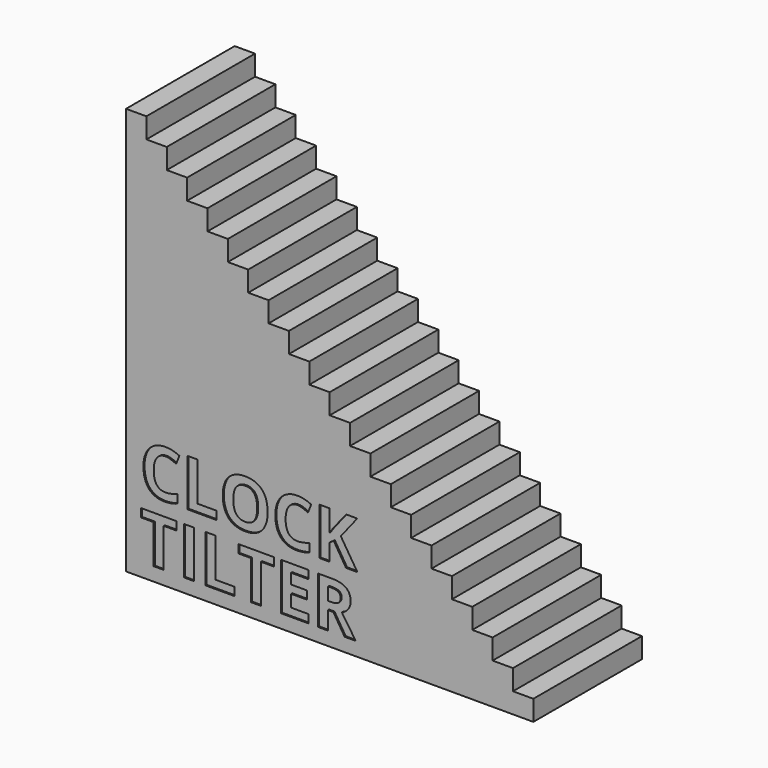
from build123d import *

# Parameters (mm, degrees)
F0_W         = 1.4720052083
F0_H         = 6.9407552083
F0_TEXT_SIZE = 9.7222222222
F1_DEPTH     = 20
F2_DEPTH     = 0.2


# Not quite as in the source:
# - Text() gives the source's letters only with a copy of the font that has no kerning and outlines rounded to 1/6400 em; it was checked with that copy


with BuildPart() as f1:
    # F0 (on Front) → F1 (new body)
    with BuildSketch(Plane.XZ):
        Polygon((-37.6443677493, -13.4150516285), (22.3556322507, -13.4150516285), (22.3556322507, -10.4150516285), (19.3556322507, -10.4150516285), (19.3556322507, -7.4150516285), (16.3556322507, -7.4150516285), (16.3556322507, -4.4150516285), (13.3556322507, -4.4150516285), (13.3556322507, -1.4150516285), (10.3556322507, -1.4150516285), (10.3556322507, 1.5849483715), (7.3556322507, 1.5849483715), (7.3556322507, 4.5849483715), (4.3556322507, 4.5849483715), (4.3556322507, 7.5849483715), (1.3556322507, 7.5849483715), (1.3556322507, 10.5849483715), (-1.6443677493, 10.5849483715), (-1.6443677493, 13.5849483715), (-4.6443677493, 13.5849483715), (-4.6443677493, 16.5849483715), (-7.6443677493, 16.5849483715), (-7.6443677493, 19.5849483715), (-10.6443677493, 19.5849483715), (-10.6443677493, 22.5849483715), (-13.6443677493, 22.5849483715), (-13.6443677493, 25.5849483715), (-16.6443677493, 25.5849483715), (-16.6443677493, 28.5849483715), (-19.6443677493, 28.5849483715), (-19.6443677493, 31.5849483715), (-22.6443677493, 31.5849483715), (-22.6443677493, 34.5849483715), (-25.6443677493, 34.5849483715), (-25.6443677493, 37.5849483715), (-28.6443677493, 37.5849483715), (-28.6443677493, 40.5849483715), (-31.6443677493, 40.5849483715), (-31.6443677493, 43.5849483715), (-34.6443677493, 43.5849483715), (-34.6443677493, 46.5849483715), (-37.6443677493, 46.5849483715), align=None)
        Polygon((-32.0927184437, -5.6986887813), (-32.0927184437, -11.4150516285), (-33.564723652, -11.4150516285), (-33.564723652, -5.6986887813), (-35.4499233048, -5.6986887813), (-35.4499233048, -4.4742964201), (-30.2090378882, -4.4742964201), (-30.2090378882, -5.6986887813), align=None, mode=Mode.SUBTRACT)
        with Locations((-28.4051099368, -7.9446740243)):
            Rectangle(F0_W, F0_H, mode=Mode.SUBTRACT)
        Polygon((-21.6352531659, -11.4150516285), (-25.922145527, -11.4150516285), (-25.922145527, -4.4742964201), (-24.4501403187, -4.4742964201), (-24.4501403187, -10.1997738507), (-21.6352531659, -10.1997738507), align=None, mode=Mode.SUBTRACT)
        with BuildLine():
            add(Edge.make_bspline(
                [(-31.049098652, 3.2625742396), (-31.4425448326, 3.4000525382), (-31.8223191382, 3.4000525382)],
                knots=[0, 0, 0, 1, 1, 1], degree=2))
            add(Edge.make_bspline(
                [(-31.8223191382, 3.4000525382), (-32.6532653187, 3.4000525382), (-33.1089944854, 2.7757035799)],
                knots=[0, 0, 0, 1, 1, 1], degree=2))
            add(Edge.make_bspline(
                [(-33.1089944854, 2.7757035799), (-33.564723652, 2.1513546215), (-33.564723652, 1.0363372604)],
                knots=[0, 0, 0, 1, 1, 1], degree=2))
            add(Edge.make_bspline(
                [(-33.564723652, 1.0363372604), (-33.564723652, -1.2848432951), (-31.8223191382, -1.2848432951)],
                knots=[0, 0, 0, 1, 1, 1], degree=2))
            add(Edge.make_bspline(
                [(-31.8223191382, -1.2848432951), (-31.0916333743, -1.2848432951), (-30.0525708743, -0.9202599618)],
                knots=[0, 0, 0, 1, 1, 1], degree=2))
            Line((-30.0525708743, -0.9202599618), (-30.0525708743, -2.1537669063))
            add(Edge.make_bspline(
                [(-30.0525708743, -2.1537669063), (-30.9063035132, -2.5107547535), (-31.9605569854, -2.5107547535)],
                knots=[0, 0, 0, 1, 1, 1], degree=2))
            add(Edge.make_bspline(
                [(-31.9605569854, -2.5107547535), (-33.4750969159, -2.5107547535), (-34.2771802493, -1.591700934)],
                knots=[0, 0, 0, 1, 1, 1], degree=2))
            add(Edge.make_bspline(
                [(-34.2771802493, -1.591700934), (-35.0792635826, -0.6726471146), (-35.0792635826, 1.0454518437)],
                knots=[0, 0, 0, 1, 1, 1], degree=2))
            add(Edge.make_bspline(
                [(-35.0792635826, 1.0454518437), (-35.0792635826, 2.1285681632), (-34.6850578534, 2.9428042743)],
                knots=[0, 0, 0, 1, 1, 1], degree=2))
            add(Edge.make_bspline(
                [(-34.6850578534, 2.9428042743), (-34.2908521243, 3.7570403854), (-33.5525708743, 4.1907426424)],
                knots=[0, 0, 0, 1, 1, 1], degree=2))
            add(Edge.make_bspline(
                [(-33.5525708743, 4.1907426424), (-32.8142896243, 4.6244448993), (-31.8223191382, 4.6244448993)],
                knots=[0, 0, 0, 1, 1, 1], degree=2))
            add(Edge.make_bspline(
                [(-31.8223191382, 4.6244448993), (-30.8121194854, 4.6244448993), (-29.791286152, 4.136814691)],
                knots=[0, 0, 0, 1, 1, 1], degree=2))
            Line((-29.791286152, 4.136814691), (-30.2652444854, 2.9397660799))
            add(Edge.make_bspline(
                [(-30.2652444854, 2.9397660799), (-30.6556524715, 3.125095941), (-31.049098652, 3.2625742396)],
                knots=[0, 0, 0, 1, 1, 1], degree=2))
        make_face(mode=Mode.SUBTRACT)
        Polygon((-24.2891160132, -2.4150516285), (-28.5760083743, -2.4150516285), (-28.5760083743, 4.5257035799), (-27.1040031659, 4.5257035799), (-27.1040031659, -1.1997738507), (-24.2891160132, -1.1997738507), align=None, mode=Mode.SUBTRACT)
        Polygon((-17.7509215687, -5.6986887813), (-17.7509215687, -11.4150516285), (-19.222926777, -11.4150516285), (-19.222926777, -5.6986887813), (-21.1081264298, -5.6986887813), (-21.1081264298, -4.4742964201), (-15.8672410132, -4.4742964201), (-15.8672410132, -5.6986887813), align=None, mode=Mode.SUBTRACT)
        Polygon((-10.8025708743, -10.1997738507), (-10.8025708743, -11.4150516285), (-14.7993156659, -11.4150516285), (-14.7993156659, -4.4742964201), (-10.8025708743, -4.4742964201), (-10.8025708743, -5.6804596146), (-13.3273104576, -5.6804596146), (-13.3273104576, -7.2041141285), (-10.9772670548, -7.2041141285), (-10.9772670548, -8.4102773229), (-13.3273104576, -8.4102773229), (-13.3273104576, -10.1997738507), align=None, mode=Mode.SUBTRACT)
        with BuildLine():
            add(Edge.make_bspline(
                [(-17.6309128882, 3.7137461146), (-16.7832566382, 2.7924136493), (-16.7832566382, 1.0652001076)],
                knots=[0, 0, 0, 1, 1, 1], degree=2))
            add(Edge.make_bspline(
                [(-16.7832566382, 1.0652001076), (-16.7832566382, -0.6589752396), (-17.6377488257, -1.5848649965)],
                knots=[0, 0, 0, 1, 1, 1], degree=2))
            add(Edge.make_bspline(
                [(-17.6377488257, -1.5848649965), (-18.4922410132, -2.5107547535), (-20.0872930965, -2.5107547535)],
                knots=[0, 0, 0, 1, 1, 1], degree=2))
            add(Edge.make_bspline(
                [(-20.0872930965, -2.5107547535), (-21.6823451798, -2.5107547535), (-22.5368373673, -1.5848649965)],
                knots=[0, 0, 0, 1, 1, 1], degree=2))
            add(Edge.make_bspline(
                [(-22.5368373673, -1.5848649965), (-23.3913295548, -0.6589752396), (-23.3913295548, 1.074314691)],
                knots=[0, 0, 0, 1, 1, 1], degree=2))
            add(Edge.make_bspline(
                [(-23.3913295548, 1.074314691), (-23.3913295548, 2.8076046215), (-22.5345587215, 3.7213416007)],
                knots=[0, 0, 0, 1, 1, 1], degree=2))
            add(Edge.make_bspline(
                [(-22.5345587215, 3.7213416007), (-21.6777878882, 4.6350785799), (-20.0781785132, 4.6350785799)],
                knots=[0, 0, 0, 1, 1, 1], degree=2))
            add(Edge.make_bspline(
                [(-20.0781785132, 4.6350785799), (-18.4785691382, 4.6350785799), (-17.6309128882, 3.7137461146)],
                knots=[0, 0, 0, 1, 1, 1], degree=2))
        make_face(mode=Mode.SUBTRACT)
        with BuildLine():
            add(Edge.make_bspline(
                [(-11.6228833743, 3.2625742396), (-12.0163295548, 3.4000525382), (-12.3961038604, 3.4000525382)],
                knots=[0, 0, 0, 1, 1, 1], degree=2))
            add(Edge.make_bspline(
                [(-12.3961038604, 3.4000525382), (-13.2270500409, 3.4000525382), (-13.6827792076, 2.7757035799)],
                knots=[0, 0, 0, 1, 1, 1], degree=2))
            add(Edge.make_bspline(
                [(-13.6827792076, 2.7757035799), (-14.1385083743, 2.1513546215), (-14.1385083743, 1.0363372604)],
                knots=[0, 0, 0, 1, 1, 1], degree=2))
            add(Edge.make_bspline(
                [(-14.1385083743, 1.0363372604), (-14.1385083743, -1.2848432951), (-12.3961038604, -1.2848432951)],
                knots=[0, 0, 0, 1, 1, 1], degree=2))
            add(Edge.make_bspline(
                [(-12.3961038604, -1.2848432951), (-11.6654180965, -1.2848432951), (-10.6263555965, -0.9202599618)],
                knots=[0, 0, 0, 1, 1, 1], degree=2))
            Line((-10.6263555965, -0.9202599618), (-10.6263555965, -2.1537669063))
            add(Edge.make_bspline(
                [(-10.6263555965, -2.1537669063), (-11.4800882354, -2.5107547535), (-12.5343417076, -2.5107547535)],
                knots=[0, 0, 0, 1, 1, 1], degree=2))
            add(Edge.make_bspline(
                [(-12.5343417076, -2.5107547535), (-14.0488816382, -2.5107547535), (-14.8509649715, -1.591700934)],
                knots=[0, 0, 0, 1, 1, 1], degree=2))
            add(Edge.make_bspline(
                [(-14.8509649715, -1.591700934), (-15.6530483048, -0.6726471146), (-15.6530483048, 1.0454518437)],
                knots=[0, 0, 0, 1, 1, 1], degree=2))
            add(Edge.make_bspline(
                [(-15.6530483048, 1.0454518437), (-15.6530483048, 2.1285681632), (-15.2588425757, 2.9428042743)],
                knots=[0, 0, 0, 1, 1, 1], degree=2))
            add(Edge.make_bspline(
                [(-15.2588425757, 2.9428042743), (-14.8646368465, 3.7570403854), (-14.1263555965, 4.1907426424)],
                knots=[0, 0, 0, 1, 1, 1], degree=2))
            add(Edge.make_bspline(
                [(-14.1263555965, 4.1907426424), (-13.3880743465, 4.6244448993), (-12.3961038604, 4.6244448993)],
                knots=[0, 0, 0, 1, 1, 1], degree=2))
            add(Edge.make_bspline(
                [(-12.3961038604, 4.6244448993), (-11.3859042076, 4.6244448993), (-10.3650708743, 4.136814691)],
                knots=[0, 0, 0, 1, 1, 1], degree=2))
            Line((-10.3650708743, 4.136814691), (-10.8390292076, 2.9397660799))
            add(Edge.make_bspline(
                [(-10.8390292076, 2.9397660799), (-11.2294371937, 3.125095941), (-11.6228833743, 3.2625742396)],
                knots=[0, 0, 0, 1, 1, 1], degree=2))
        make_face(mode=Mode.SUBTRACT)
        with BuildLine():
            Line((-7.1005309437, -8.7520741979), (-7.8828660132, -8.7520741979))
            Line((-7.8828660132, -8.7520741979), (-7.8828660132, -11.4150516285))
            Line((-7.8828660132, -11.4150516285), (-9.3548712215, -11.4150516285))
            Line((-9.3548712215, -11.4150516285), (-9.3548712215, -4.4742964201))
            Line((-9.3548712215, -4.4742964201), (-7.3329528187, -4.4742964201))
            add(Edge.make_bspline(
                [(-7.3329528187, -4.4742964201), (-5.9171542076, -4.4742964201), (-5.2388772979, -4.9892703785)],
                knots=[0, 0, 0, 1, 1, 1], degree=2))
            add(Edge.make_bspline(
                [(-5.2388772979, -4.9892703785), (-4.5606003882, -5.5042443368), (-4.5606003882, -6.5539405174)],
                knots=[0, 0, 0, 1, 1, 1], degree=2))
            add(Edge.make_bspline(
                [(-4.5606003882, -6.5539405174), (-4.5606003882, -7.1661366979), (-4.8970804229, -7.6431332257)],
                knots=[0, 0, 0, 1, 1, 1], degree=2))
            add(Edge.make_bspline(
                [(-4.8970804229, -7.6431332257), (-5.2335604576, -8.1201297535), (-5.851833027, -8.390529059)],
                knots=[0, 0, 0, 1, 1, 1], degree=2))
            add(Edge.make_bspline(
                [(-5.851833027, -8.390529059), (-4.2841246937, -10.7314578785), (-3.8101663604, -11.4150516285)],
                knots=[0, 0, 0, 1, 1, 1], degree=2))
            Line((-3.8101663604, -11.4150516285), (-5.4431958743, -11.4150516285))
            Line((-5.4431958743, -11.4150516285), (-7.1005309437, -8.7520741979))
        make_face(mode=Mode.SUBTRACT)
        Polygon((-6.0067809437, 1.4540889965), (-3.5671108048, -2.4150516285), (-5.2381177493, -2.4150516285), (-7.0564771243, 0.5092105243), (-7.6777878882, 0.062595941), (-7.6777878882, -2.4150516285), (-9.1497930965, -2.4150516285), (-9.1497930965, 4.5257035799), (-7.6777878882, 4.5257035799), (-7.6777878882, 1.3492712882), (-7.0990118465, 2.1665455937), (-5.2183694854, 4.5257035799), (-3.5853399715, 4.5257035799), align=None, mode=Mode.SUBTRACT)
        with BuildLine():
            add(Edge.make_bspline(
                [(-21.4020717423, 2.8182383021), (-21.847926777, 2.2273094826), (-21.847926777, 1.0652001076)],
                knots=[0, 0, 0, 1, 1, 1], degree=2))
            add(Edge.make_bspline(
                [(-21.847926777, 1.0652001076), (-21.847926777, -0.0984283646), (-21.406629034, -0.6870785382)],
                knots=[0, 0, 0, 1, 1, 1], degree=2))
            add(Edge.make_bspline(
                [(-21.406629034, -0.6870785382), (-20.9653312909, -1.2757287118), (-20.0872930965, -1.2757287118)],
                knots=[0, 0, 0, 1, 1, 1], degree=2))
            add(Edge.make_bspline(
                [(-20.0872930965, -1.2757287118), (-18.3266594159, -1.2757287118), (-18.3266594159, 1.0652001076)],
                knots=[0, 0, 0, 1, 1, 1], degree=2))
            add(Edge.make_bspline(
                [(-18.3266594159, 1.0652001076), (-18.3266594159, 3.4091671215), (-20.0781785132, 3.4091671215)],
                knots=[0, 0, 0, 1, 1, 1], degree=2))
            add(Edge.make_bspline(
                [(-20.0781785132, 3.4091671215), (-20.9562167076, 3.4091671215), (-21.4020717423, 2.8182383021)],
                knots=[0, 0, 0, 1, 1, 1], degree=2))
        make_face()
        with Locations((-35.6443677493, -2.4150516285)):
            Text('CLOCK', F0_TEXT_SIZE, font='Open Sans', font_style=FontStyle.BOLD, text_align=(TextAlign.LEFT, TextAlign.BOTTOM))
        with Locations((-35.6443677493, -11.4150516285)):
            Text('TILTER', F0_TEXT_SIZE, font='Open Sans', font_style=FontStyle.BOLD, text_align=(TextAlign.LEFT, TextAlign.BOTTOM))
        with BuildLine():
            Line((-7.8828660132, -5.6804596146), (-7.8828660132, -7.5550255868))
            Line((-7.8828660132, -7.5550255868), (-7.4089076798, -7.5550255868))
            add(Edge.make_bspline(
                [(-7.4089076798, -7.5550255868), (-6.7101229576, -7.5550255868), (-6.3782002145, -7.3226037118)],
                knots=[0, 0, 0, 1, 1, 1], degree=2))
            add(Edge.make_bspline(
                [(-6.3782002145, -7.3226037118), (-6.0462774715, -7.0901818368), (-6.0462774715, -6.5919179479)],
                knots=[0, 0, 0, 1, 1, 1], degree=2))
            add(Edge.make_bspline(
                [(-6.0462774715, -6.5919179479), (-6.0462774715, -6.0982113507), (-6.3857957007, -5.8893354826)],
                knots=[0, 0, 0, 1, 1, 1], degree=2))
            add(Edge.make_bspline(
                [(-6.3857957007, -5.8893354826), (-6.7253139298, -5.6804596146), (-7.4362514298, -5.6804596146)],
                knots=[0, 0, 0, 1, 1, 1], degree=2))
            Line((-7.4362514298, -5.6804596146), (-7.8828660132, -5.6804596146))
        make_face()
    extrude(amount=-F1_DEPTH)

    # F0 (on Front) → F2 (cut)
    with BuildSketch(Plane.XZ):
        with Locations((-35.6443677493, -2.4150516285)):
            Text('CLOCK', F0_TEXT_SIZE, font='Open Sans', font_style=FontStyle.BOLD, text_align=(TextAlign.LEFT, TextAlign.BOTTOM))
        with Locations((-35.6443677493, -11.4150516285)):
            Text('TILTER', F0_TEXT_SIZE, font='Open Sans', font_style=FontStyle.BOLD, text_align=(TextAlign.LEFT, TextAlign.BOTTOM))
    extrude(amount=-F2_DEPTH, mode=Mode.SUBTRACT)


solid = f1.part
